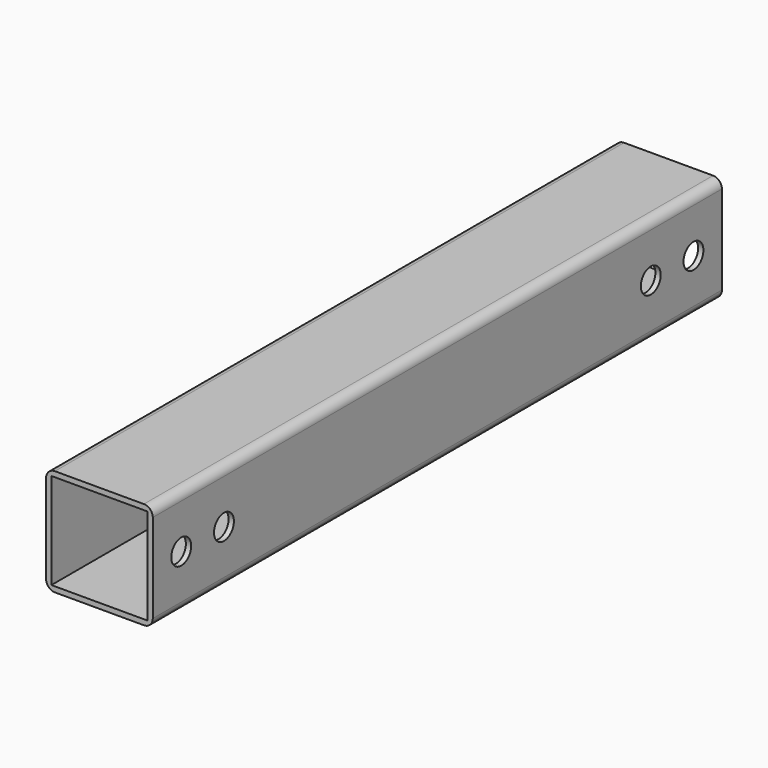
from build123d import *

# Parameters (mm, degrees)
F0_W     = 54
F0_H     = 54
F1_DEPTH = 400
F2_R     = 7
F3_DEPTH = 3


# Not quite as in the source:
# - a feature names something its author has since deleted; it is built from what else it names


with BuildPart() as f1:
    # F0 (on Front) → F1 (new body)
    with BuildSketch(Plane.XZ):
        with BuildLine():
            ThreePointArc((-28.9867345989, -60.995567819), (-30.4512006929, -57.460033913), (-33.9867345989, -55.995567819))
            Line((-33.9867345989, -55.995567819), (-83.9867345989, -55.995567819))
            ThreePointArc((-83.9867345989, -55.995567819), (-87.5222685048, -57.460033913), (-88.9867345989, -60.995567819))
            Line((-88.9867345989, -60.995567819), (-88.9867345989, -110.995567819))
            ThreePointArc((-88.9867345989, -110.995567819), (-87.5222685048, -114.5311017249), (-83.9867345989, -115.995567819))
            Line((-83.9867345989, -115.995567819), (-33.9867345989, -115.995567819))
            ThreePointArc((-33.9867345989, -115.995567819), (-30.4512006929, -114.5311017249), (-28.9867345989, -110.995567819))
            Line((-28.9867345989, -110.995567819), (-28.9867345989, -60.995567819))
        make_face()
        with Locations((-58.9867345989, -85.995567819)):
            Rectangle(F0_W, F0_H, mode=Mode.SUBTRACT)
    extrude(amount=-F1_DEPTH)

    # F2 (on face) → F3 (cut, through all)
    with BuildSketch(Plane.YZ.offset(-28.9867345989)):
        with Locations((20, -85.995567819)):
            Circle(F2_R)
        with Locations((50, -85.995567819)):
            Circle(F2_R)
        with Locations((350, -85.995567819)):
            Circle(F2_R)
        with Locations((380, -85.995567819)):
            Circle(F2_R)
    extrude(amount=-F3_DEPTH, mode=Mode.SUBTRACT)


solid = f1.part
